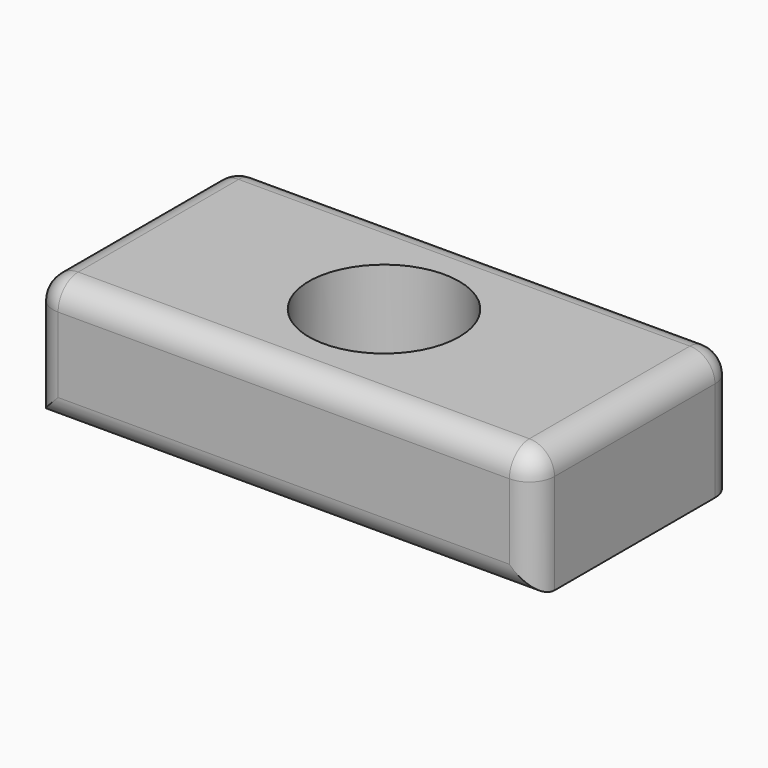
from build123d import *

# Parameters (mm, degrees)
F0_W        = 100
F0_H        = 50
F1_DEPTH    = 25
F2_R        = 15
F3_DEPTH    = 25.001
F4_R        = 5
F5_T1_DEPTH = 32.5
F5_S5_W     = 5
F5_S5_H     = 5
F5_T6_DEPTH = 5
F6_T1_DEPTH = 32.5
F6_S5_W     = 5
F6_S5_H     = 5
F6_T6_DEPTH = 5


# Not quite as in the source:
# - a fillet or chamfer that OpenCascade refuses, or shapes differently, is made with other operations: its cross-section is extruded or revolved along the edge and cut away or added


with BuildPart() as f1:
    # F0 (on Top) → F1 (new body)
    with BuildSketch(Plane.XY):
        Rectangle(F0_W, F0_H)
    extrude(amount=F1_DEPTH)

    # F2 (on face) → F3 (cut, through all)
    with BuildSketch(Plane.XY.offset(25)):
        Circle(F2_R)
    extrude(amount=-F3_DEPTH, mode=Mode.SUBTRACT)

    # F4
    f4_edges = [f1.edges().sort_by_distance(p)[0] for p in [
        (0, 25, 25),
        (-50, 0, 25),
        (-50, -25, 12.5),
        (50, -25, 12.5),
        (0, -25, 0),
        (0, -25, 25),
        (50, 0, 25),
    ]]
    fillet(f4_edges, radius=F4_R)

    # F5: fillet of radius 5 on 1 edges, made by hand

    # F5_s2 → F5_t1 (cut)
    with BuildSketch(Plane.XY.offset(-12.5)):
        with BuildLine():
            ThreePointArc((-50, 20), (-48.5355339059, 23.5355339059), (-45, 25))
            Line((-45, 25), (-50, 25))
            Line((-50, 25), (-50, 20))
        make_face()
    extrude(amount=F5_T1_DEPTH, mode=Mode.SUBTRACT)


with BuildPart() as f5_tool4:
    # F5_s5 → F5_t6 (new body)
    with BuildSketch(Plane.YZ.offset(-45)):
        with Locations((22.5, 22.5)):
            Rectangle(F5_S5_W, F5_S5_H)
    extrude(amount=-F5_T6_DEPTH)

    # F5_s7 → F5_t8 (revolve, cut)
    with BuildSketch(Plane(origin=(-45, 20, 20), x_dir=(0, -0.7071067812, -0.7071067812), z_dir=(0, 0.7071067812, -0.7071067812))):
        with BuildLine():
            ThreePointArc((0, -5), (5, 0), (0, 5))
            Line((0, 5), (0, -5))
        make_face()
    revolve(axis=Axis((-45, 20, 20), (-1, 0, 0)), mode=Mode.SUBTRACT)


with BuildPart() as f1_1:
    add(f1.part)

    # F5_t3: cut F5_tool4
    add(f5_tool4.part, mode=Mode.SUBTRACT)

    # F6: fillet of radius 5 on 1 edges, made by hand

    # F6_s2 → F6_t1 (cut)
    with BuildSketch(Plane.XY.offset(-12.5)):
        with BuildLine():
            ThreePointArc((45, 25), (48.5355339059, 23.5355339059), (50, 20))
            Line((50, 20), (50, 25))
            Line((50, 25), (45, 25))
        make_face()
    extrude(amount=F6_T1_DEPTH, mode=Mode.SUBTRACT)


with BuildPart() as f6_tool4:
    # F6_s5 → F6_t6 (new body)
    with BuildSketch(Plane.XZ.offset(-20)):
        with Locations((47.5, 22.5)):
            Rectangle(F6_S5_W, F6_S5_H)
    extrude(amount=-F6_T6_DEPTH)

    # F6_s7 → F6_t8 (revolve, cut)
    with BuildSketch(Plane(origin=(45, 20, 20), x_dir=(-0.7071067812, 0, -0.7071067812), z_dir=(0.7071067812, 0, -0.7071067812))):
        with BuildLine():
            ThreePointArc((0, -5), (5, 0), (0, 5))
            Line((0, 5), (0, -5))
        make_face()
    revolve(axis=Axis((45, 20, 20), (0, 1, 0)), mode=Mode.SUBTRACT)


with BuildPart() as f1_2:
    add(f1_1.part)

    # F6_t3: cut F6_tool4
    add(f6_tool4.part, mode=Mode.SUBTRACT)


solid = f1_2.part
